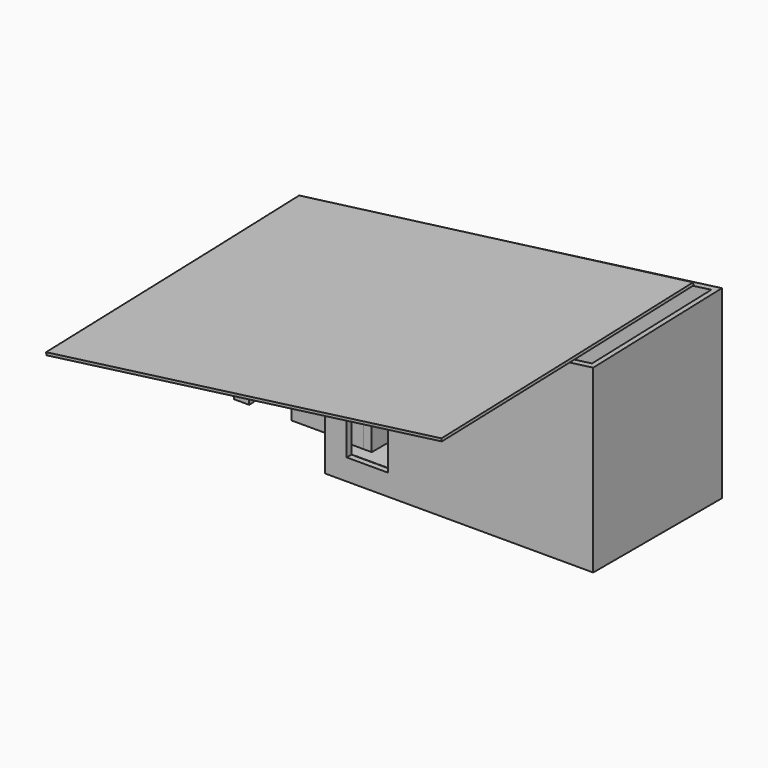
from build123d import *

# Parameters (mm, degrees)
F7_DEPTH  = 50
F8_REACH  = 9267.0421515008
F9_W      = 792.9490208626
F9_H      = 1923.7364530563
F10_DEPTH = 110
F11_W     = 773.6711502075
F11_H     = 1769.0812349319
F12_DEPTH = 110
F13_DEPTH = 400
F14_W     = 660
F14_H     = 790
F15_DEPTH = 480
F14_H_2   = 810
F16_DEPTH = 330
F17_W     = 2000
F17_H     = 1500
F18_DEPTH = 1500
F17_W_2   = 1000
F19_DEPTH = 1000
F20_W     = 2500
F20_H     = 50
F21_DEPTH = 600


# Not quite as in the source:
# - a feature names something its author has since deleted; it is built from what else it names


with BuildPart() as f7:
    # F6 (on 3pt) → F7 (new body)
    with BuildSketch(Plane(origin=(-321.5081857629, -69.1366251757, 2411.3113932214), x_dir=(0.9912350116, -0.0037862856, 0.1320561086), z_dir=(0.1321103773, 0.0284088121, -0.9908278295))):
        Polygon((-62.647297173, 173.9513684009), (-70.2198684375, -1825.2270662935), (2407.8676605606, -1825.2270662935), (7364.0427185569, -1825.2270662935), (7375.4015754536, 1173.5405857481), (7375.4015754536, 4057.758942678), (-62.647297173, 4085.9330937089), align=None)
    extrude(amount=F7_DEPTH)


with BuildPart() as f8:
    f8_end = Plane(origin=(3304.4233440469, -1204.757655027, 2811.745783625), x_dir=(-0.9912279007, 0, -0.1321637201), z_dir=(0.1321103773, 0.0284088121, -0.9908278295))
    # F0 (on Top) → F8 (new body, up to a plane its end follows)
    with BuildSketch(Plane.XY):
        Polygon((7436.1340180039, 1825.9771460295), (2436.1340180039, 1825.9771460295), (2436.1340180039, 1715.9771460295), (2436.1340180039, 1404.0166139603), (2546.1340180039, 1404.0166139603), (2546.1340180039, 1715.9771460295), (7326.1340180039, 1715.9771460295), (7326.1340180039, -1064.0228539705), (2546.1340180039, -1064.0228539705), (2546.1340180039, 217.7686989307), (2436.1340180039, 217.7686989307), (2436.1340180039, -64.0228539705), (2436.1340180039, -174.0228539705), (2436.1340180039, -1174.0228539705), (7436.1340180039, -1174.0228539705), align=None)
        Polygon((2436.1340180039, 1825.9771460295), (-63.8659819961, 1825.9771460295), (-63.8659819961, -174.0228539705), (2436.1340180039, -174.0228539705), (2436.1340180039, -64.0228539705), (46.1340180039, -64.0228539705), (46.1340180039, 1715.9771460295), (2436.1340180039, 1715.9771460295), align=None)
    f8_long = extrude(amount=F8_REACH, mode=Mode.PRIVATE)
    add(split(f8_long, bisect_by=f8_end, keep=Keep.TOP, mode=Mode.PRIVATE))

    # F9 (on face) → F10 (cut, through all)
    with BuildSketch(Plane.XZ.offset(174.0228539705)):
        with Locations((615.8994138241, 961.8682265282)):
            Rectangle(F9_W, F9_H)
    extrude(amount=-F10_DEPTH, mode=Mode.SUBTRACT)

    # F11 (on face) → F12 (cut, through all)
    with BuildSketch(Plane.XZ.offset(1174.0228539705)):
        with Locations((3224.5798110962, 1279.4668078423)):
            Rectangle(F11_W, F11_H)
    extrude(amount=-F12_DEPTH, mode=Mode.SUBTRACT)

    # F0 (on Top) → F13 (join)
    with BuildSketch(Plane.XY):
        Polygon((2546.1340180039, 1715.9771460295), (2546.1340180039, 1404.0166139603), (2546.1340180039, 217.7686989307), (2546.1340180039, -1064.0228539705), (7326.1340180039, -1064.0228539705), (7326.1340180039, 1715.9771460295), align=None)
    extrude(amount=F13_DEPTH)


with BuildPart() as f15:
    # F14 (on face) → F15 (new body)
    with BuildSketch(Plane.YZ.offset(2546.1340180039)):
        with Locations((-494.0228539705, 795)):
            Rectangle(F14_W, F14_H)
    extrude(amount=F15_DEPTH)


with BuildPart() as f16:
    # F14 (on face) → F16 (new body)
    with BuildSketch(Plane.YZ.offset(2546.1340180039)):
        with Locations((-494.0228539705, 795)):
            Rectangle(F14_W, F14_H)
        with Locations((-494.0228539705, 1595)):
            Rectangle(F14_W, F14_H_2)
    extrude(amount=F16_DEPTH)


with BuildPart() as f18:
    # F17 (on face) → F18 (new body)
    with BuildSketch(Plane.XY.offset(400)):
        with Locations((3846.1340180039, 665.9771460295)):
            Rectangle(F17_W, F17_H)
    extrude(amount=F18_DEPTH)


with BuildPart() as f19:
    # F17 (on face) → F19 (new body)
    with BuildSketch(Plane.XY.offset(400)):
        with Locations((5346.1340180039, 665.9771460295)):
            Rectangle(F17_W_2, F17_H)
    extrude(amount=F19_DEPTH)


with BuildPart() as f21:
    # F20 (on face) → F21 (new body)
    with BuildSketch(Plane(origin=(0, -1064.0228539705, 0), x_dir=(-1, 0, 0), z_dir=(0, 1, 0))):
        with Locations((-4861.4153862, 1425)):
            Rectangle(F20_W, F20_H)
    extrude(amount=F21_DEPTH)


solid = Compound([f7.part, f8.part, f15.part, f16.part, f18.part, f19.part, f21.part])
